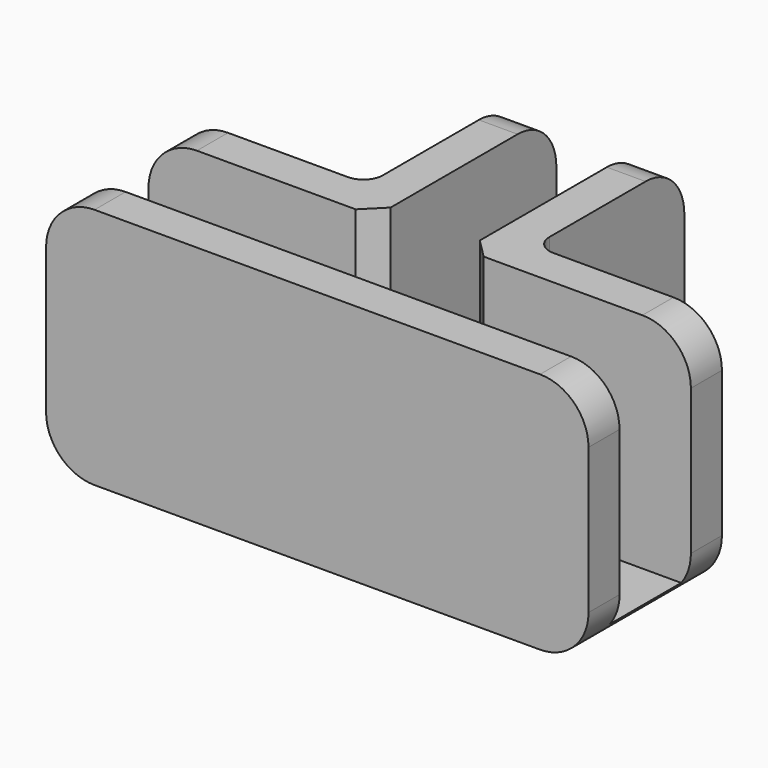
from build123d import *

# Parameters (mm, degrees)
F1_DEPTH       = 2
F2_DEPTH       = 25
F3_R           = 2
F4_T1_DEPTH    = 29
F4_T3_DEPTH    = 29
F4_T5_DEPTH    = 29
F4_T7_DEPTH    = 29
F4_T9_DEPTH    = 42.2
F4_T11_DEPTH   = 42.2
F5_R           = 2
F6_SIZE        = 2
F8_D           = 3.3
F8_CSINK_D     = 6
F8_CSINK_ANGLE = 90


# Not quite as in the source:
# - a fillet or chamfer that OpenCascade refuses, or shapes differently, is made with other operations: its cross-section is extruded or revolved along the edge and cut away or added


with BuildPart() as f1:
    # F0 (on Top) → F1 (new body)
    with BuildSketch(Plane.XY):
        Polygon((-27.6520505063, 0), (0, 0), (28.2951036699, 0), (28.2951036699, 9.2), (4.9215265818, 9.2), (4.9215265818, 32.5735770881), (-4.2784734182, 32.5735770881), (-4.2784734182, 9.2), (-27.6520505063, 9.2), align=None)
        Polygon((28.2951036699, 0), (0, 0), (-27.6520505063, 0), (-27.6520505063, -4), (0, -4), (28.2951036699, -4), align=None)
        Polygon((4.9215265818, 9.2), (28.2951036699, 9.2), (28.2951036699, 13.2), (8.9215265818, 13.2), (8.9215265818, 32.5735770881), (4.9215265818, 32.5735770881), align=None)
        Polygon((-27.6520505063, 13.2), (-27.6520505063, 9.2), (-4.2784734182, 9.2), (-4.2784734182, 32.5735770881), (-8.2784734182, 32.5735770881), (-8.2784734182, 13.2), align=None)
    extrude(amount=F1_DEPTH)

    # F0 (on Top) → F2 (join)
    with BuildSketch(Plane.XY):
        Polygon((-27.6520505063, 13.2), (-27.6520505063, 9.2), (-4.2784734182, 9.2), (-4.2784734182, 32.5735770881), (-8.2784734182, 32.5735770881), (-8.2784734182, 13.2), align=None)
        Polygon((4.9215265818, 9.2), (28.2951036699, 9.2), (28.2951036699, 13.2), (8.9215265818, 13.2), (8.9215265818, 32.5735770881), (4.9215265818, 32.5735770881), align=None)
        Polygon((28.2951036699, 0), (0, 0), (-27.6520505063, 0), (-27.6520505063, -4), (0, -4), (28.2951036699, -4), align=None)
    extrude(amount=F2_DEPTH)

    # F3
    f3_edges = [f1.edges().sort_by_distance(p)[0] for p in [
        (8.921527, 13.2, 12.5),
    ]]
    fillet(f3_edges, radius=F3_R)

    # F4: fillet of radius 5 on 9 edges, made by hand

    # F4_s2 → F4_t1 (cut)
    with BuildSketch(Plane.XZ.offset(-12.5)):
        with BuildLine():
            ThreePointArc((28.2951036699, 20), (26.8306375758, 23.5355339059), (23.2951036699, 25))
            Line((23.2951036699, 25), (28.2951036699, 25))
            Line((28.2951036699, 25), (28.2951036699, 20))
        make_face()
        with BuildLine():
            ThreePointArc((-27.6520505063, 20), (-26.1875844123, 23.5355339059), (-22.6520505063, 25))
            Line((-22.6520505063, 25), (-27.6520505063, 25))
            Line((-27.6520505063, 25), (-27.6520505063, 20))
        make_face()
    extrude(amount=F4_T1_DEPTH, mode=Mode.SUBTRACT)

    # F4_s4 → F4_t3 (cut)
    with BuildSketch(Plane.XZ.offset(-25.7)):
        with BuildLine():
            ThreePointArc((28.2951036699, 20), (26.8306375758, 23.5355339059), (23.2951036699, 25))
            Line((23.2951036699, 25), (28.2951036699, 25))
            Line((28.2951036699, 25), (28.2951036699, 20))
        make_face()
        with BuildLine():
            ThreePointArc((-27.6520505063, 20), (-26.1875844123, 23.5355339059), (-22.6520505063, 25))
            Line((-22.6520505063, 25), (-27.6520505063, 25))
            Line((-27.6520505063, 25), (-27.6520505063, 20))
        make_face()
    extrude(amount=F4_T3_DEPTH, mode=Mode.SUBTRACT)

    # F4_s6 → F4_t5 (cut)
    with BuildSketch(Plane.YZ.offset(-20.7784734182)):
        with BuildLine():
            ThreePointArc((32.5735770881, 20), (31.1091109941, 23.5355339059), (27.5735770881, 25))
            Line((27.5735770881, 25), (32.5735770881, 25))
            Line((32.5735770881, 25), (32.5735770881, 20))
        make_face()
    extrude(amount=F4_T5_DEPTH, mode=Mode.SUBTRACT)

    # F4_s8 → F4_t7 (cut)
    with BuildSketch(Plane.YZ.offset(-7.5784734182)):
        with BuildLine():
            ThreePointArc((32.5735770881, 20), (31.1091109941, 23.5355339059), (27.5735770881, 25))
            Line((27.5735770881, 25), (32.5735770881, 25))
            Line((32.5735770881, 25), (32.5735770881, 20))
        make_face()
    extrude(amount=F4_T7_DEPTH, mode=Mode.SUBTRACT)

    # F4_s10 → F4_t9 (cut)
    with BuildSketch(Plane.XZ.offset(-25.7)):
        with BuildLine():
            ThreePointArc((-22.6520505063, 0), (-26.1875844123, 1.4644660941), (-27.6520505063, 5))
            Line((-27.6520505063, 5), (-27.6520505063, 0))
            Line((-27.6520505063, 0), (-22.6520505063, 0))
        make_face()
        with BuildLine():
            ThreePointArc((23.2951036699, 0), (26.8306375758, 1.4644660941), (28.2951036699, 5))
            Line((28.2951036699, 5), (28.2951036699, 0))
            Line((28.2951036699, 0), (23.2951036699, 0))
        make_face()
    extrude(amount=F4_T9_DEPTH, mode=Mode.SUBTRACT)

    # F4_s12 → F4_t11 (cut)
    with BuildSketch(Plane.YZ.offset(-20.7784734182)):
        with BuildLine():
            ThreePointArc((27.5735770881, 0), (31.1091109941, 1.4644660941), (32.5735770881, 5))
            Line((32.5735770881, 5), (32.5735770881, 0))
            Line((32.5735770881, 0), (27.5735770881, 0))
        make_face()
    extrude(amount=F4_T11_DEPTH, mode=Mode.SUBTRACT)

    # F5
    f5_edges = [f1.edges().sort_by_distance(p)[0] for p in [
        (-8.278473, 13.2, 12.5),
    ]]
    fillet(f5_edges, radius=F5_R)

    # F6
    f6_edges = [f1.edges().sort_by_distance(p)[0] for p in [
        (4.921527, 9.2, 13.5),
        (-4.278473, 9.2, 13.5),
    ]]
    chamfer(f6_edges, length=F6_SIZE)

    # F8 (through all)
    with Locations(Plane(origin=(0, 0, 0), x_dir=(1, 0, 0), z_dir=(0, 0, -1))):
        with Locations((-15, -4.6), (0, -19.6), (15, -4.6)):
            CounterSinkHole(F8_D / 2, F8_CSINK_D / 2, counter_sink_angle=F8_CSINK_ANGLE)


solid = f1.part
